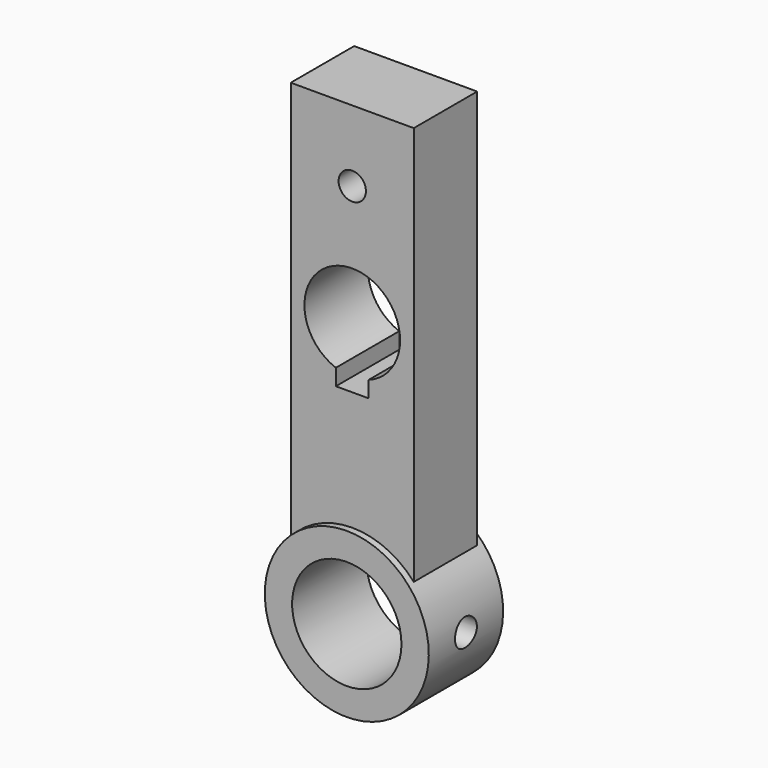
from build123d import *

# Parameters (mm, degrees)
F0_R     = 20
F1_DEPTH = 17
F2_R     = 5
F3_DEPTH = 30.001
F4_DEPTH = 12.5
F0_R_2   = 5
F5_DEPTH = 14.5


# Not quite as in the source:
# - a feature names something its author has since deleted; it is built from what else it names


with BuildPart() as f1:
    # F0 (on Front) → F1 (new body, symmetric)
    with BuildSketch(Plane.XZ):
        with BuildLine():
            ThreePointArc((-22.5, 19.843134833), (-10.6066017178, -28.0624304008), (30, 0))
            ThreePointArc((30, 0), (28.0624304008, 10.6066017178), (22.5, 19.843134833))
            ThreePointArc((22.5, 19.843134833), (0, 30), (-22.5, 19.843134833))
        make_face()
        Circle(F0_R, mode=Mode.SUBTRACT)
    extrude(amount=F1_DEPTH, both=True)

    # F2 (on Right) → F3 (cut, through all)
    with BuildSketch(Plane.YZ):
        Circle(F2_R)
    extrude(amount=F3_DEPTH, mode=Mode.SUBTRACT)

    # F0 (on Front) → F4 (cut, symmetric)
    with BuildSketch(Plane.XZ):
        with BuildLine():
            ThreePointArc((6, 79.5607177772), (0, 78.5), (-6, 79.5607177772))
            Line((-6, 79.5607177772), (-6, 73.6))
            Line((-6, 73.6), (6, 73.6))
            Line((6, 73.6), (6, 79.5607177772))
        make_face()
    extrude(amount=F4_DEPTH, both=True, mode=Mode.SUBTRACT)

    # F0 (on Front) → F5 (join, symmetric)
    with BuildSketch(Plane.XZ):
        with BuildLine():
            ThreePointArc((-22.5, 19.843134833), (0, 30), (22.5, 19.843134833))
            Line((22.5, 19.843134833), (22.5, 166))
            Line((22.5, 166), (-22.5, 166))
            Line((-22.5, 166), (-22.5, 19.843134833))
        make_face()
        with BuildLine():
            ThreePointArc((-6, 79.5607177772), (-10.0312013239, 110.3396303997), (17.5, 96))
            ThreePointArc((17.5, 96), (14.3396303997, 85.9687986761), (6, 79.5607177772))
            Line((6, 79.5607177772), (6, 73.6))
            Line((6, 73.6), (-6, 73.6))
            Line((-6, 73.6), (-6, 79.5607177772))
        make_face(mode=Mode.SUBTRACT)
        with Locations((0, 140)):
            Circle(F0_R_2, mode=Mode.SUBTRACT)
    extrude(amount=F5_DEPTH, both=True)


solid = f1.part
